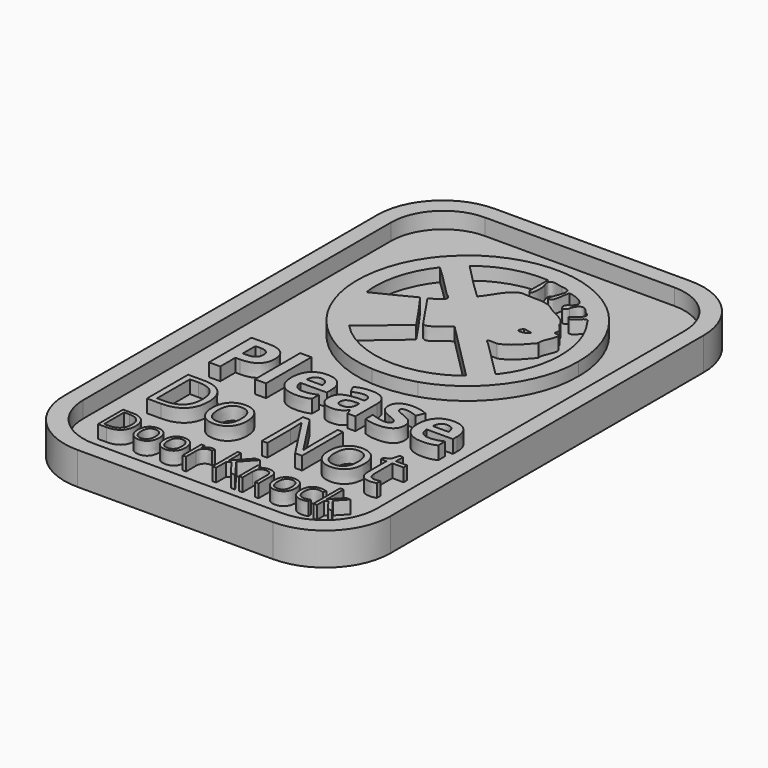
from build123d import *

# Parameters (mm, degrees)
F0_W           = 50
F0_H           = 25
F0_H_2         = 55
F1_DEPTH       = 5
F2_T           = -2.5
F3_TEXT_SIZE   = 11.4280198832
F3_TEXT_SIZE_2 = 11.0519929058
F3_TEXT_SIZE_3 = 6.7370337705
F4_DEPTH       = 2
F5_R           = 8
F6_R           = 10
F8_DEPTH       = 2


# Not quite as in the source:
# - ends of sketch curves that miss each other by under 0.0002 mm in the source are joined
# - Text() gives the source's letters only with a copy of the font that has no kerning and outlines rounded to 1/6400 em; it was checked with that copy


with BuildPart() as f1:
    # F0 (on Top) → F1 (new body)
    with BuildSketch(Plane.XY):
        with Locations((0, 12.5)):
            Rectangle(F0_W, F0_H)
        with Locations((0, -27.5)):
            Rectangle(F0_W, F0_H_2)
    extrude(amount=F1_DEPTH)

    # F2
    f2_openings = [f1.faces().sort_by_distance(p)[0] for p in [
        (0, -15, 5),
    ]]
    offset(amount=F2_T, openings=f2_openings)

    # F3 (on face) → F4 (join)
    with BuildSketch(Plane.XY.offset(2.5)):
        with Locations((-18.5, -26.691900793)):
            Text('Please', F3_TEXT_SIZE, font='Open Sans', font_style=FontStyle.BOLD, text_align=(TextAlign.LEFT, TextAlign.BOTTOM))
        with Locations((-18.5, -38.6493356852)):
            Text('Do Not', F3_TEXT_SIZE_2, font='Open Sans', text_align=(TextAlign.LEFT, TextAlign.BOTTOM))
        with Locations((-18.5, -47.5)):
            Text('Door Knock', F3_TEXT_SIZE_3, font='Open Sans', text_align=(TextAlign.LEFT, TextAlign.BOTTOM))
    extrude(amount=F4_DEPTH)

    # F5
    f5_edges = [f1.edges().sort_by_distance(p)[0] for p in [
        (-22.5, 22.5, 3.75),
        (22.5, 22.5, 3.75),
        (22.5, -52.5, 3.75),
        (-22.5, -52.5, 3.75),
    ]]
    fillet(f5_edges, radius=F5_R)

    # F6
    f6_edges = [f1.edges().sort_by_distance(p)[0] for p in [
        (-25, 25, 2.5),
        (-25, -55, 2.5),
        (25, -55, 2.5),
        (25, 25, 2.5),
    ]]
    fillet(f6_edges, radius=F6_R)

    # F7 (on face) → F8 (join)
    with BuildSketch(Plane.XY.offset(2.5)):
        with BuildLine():
            add(Edge.make_bspline(
                [(-1.152975, -15.828035), (-7.683402, -15.45201), (-13.720566, -10.924744), (-15.897689, -4.754124)],
                knots=[0, 0, 0, 0, 1, 1, 1, 1], degree=3))
            add(Edge.make_bspline(
                [(5.254472, -15.031673), (3.193987, -15.71671), (1.009548, -15.937421), (-1.152975, -15.828035)],
                knots=[0, 0, 0, 0, 1, 1, 1, 1], degree=3))
            add(Edge.make_bspline(
                [(16.918267, 1.099339), (17.077182, -6.063448), (12.07656, -12.904762), (5.254472, -15.031673)],
                knots=[0, 0, 0, 0, 1, 1, 1, 1], degree=3))
            add(Edge.make_bspline(
                [(6.093725, 16.862866), (12.482614, 14.48419), (17.023863, 7.927673), (16.918267, 1.099339)],
                knots=[0, 0, 0, 0, 1, 1, 1, 1], degree=3))
            add(Edge.make_bspline(
                [(-12.087027, 12.911491), (-7.523079, 17.697854), (-0.044603, 19.290758), (6.093725, 16.862866)],
                knots=[0, 0, 0, 0, 1, 1, 1, 1], degree=3))
            add(Edge.make_bspline(
                [(-15.897689, -4.754124), (-18.132821, 1.226539), (-16.624786, 8.400491), (-12.087027, 12.911491)],
                knots=[0, 0, 0, 0, 1, 1, 1, 1], degree=3))
        make_face()
        with BuildLine():
            add(Edge.make_bspline(
                [(1.660306, -13.112709), (4.218505, -12.787149), (6.73921, -11.822528), (8.738555, -10.17936)],
                knots=[0, 0, 0, 0, 1, 1, 1, 1], degree=3))
            add(Edge.make_bspline(
                [(-10.297667, -8.802453), (-7.267469, -12.026995), (-2.724918, -13.624278), (1.660306, -13.112709)],
                knots=[0, 0, 0, 0, 1, 1, 1, 1], degree=3))
            add(Edge.make_bspline(
                [(-4.186312, -3.599084), (-6.159197, -5.403336), (-8.265193, -7.063118), (-10.297667, -8.802453)],
                knots=[0, 0, 0, 0, 1, 1, 1, 1], degree=3))
            add(Edge.make_bspline(
                [(-8.239712, 2.231822), (-6.846707, 0.318469), (-5.495582, -1.627468), (-4.186312, -3.599084)],
                knots=[0, 0, 0, 0, 1, 1, 1, 1], degree=3))
            add(Edge.make_bspline(
                [(-14.12669, -0.727469), (-12.153893, 0.147058), (-10.217288, 1.29033), (-8.239712, 2.231822)],
                knots=[0, 0, 0, 0, 1, 1, 1, 1], degree=3))
            add(Edge.make_bspline(
                [(-11.252573, 9.780323), (-13.58058, 6.880246), (-14.657997, 2.956887), (-14.12669, -0.727469)],
                knots=[0, 0, 0, 0, 1, 1, 1, 1], degree=3))
            add(Edge.make_bspline(
                [(-6.241496, 4.836455), (-7.914058, 6.474699), (-9.527901, 8.223918), (-11.252573, 9.780323)],
                knots=[0, 0, 0, 0, 1, 1, 1, 1], degree=3))
            add(Edge.make_bspline(
                [(-7.363937, 2.526994), (-6.492223, 3.287102), (-4.519532, 3.854826), (-6.241496, 4.836455)],
                knots=[0, 0, 0, 0, 1, 1, 1, 1], degree=3))
            add(Edge.make_bspline(
                [(-3.768493, -2.787968), (-4.965583, -1.015428), (-6.195906, 0.735116), (-7.363937, 2.526994)],
                knots=[0, 0, 0, 0, 1, 1, 1, 1], degree=3))
            add(Edge.make_bspline(
                [(-0.275679, -1.122884), (-1.382058, -1.544562), (-2.812765, -3.748359), (-3.768493, -2.787968)],
                knots=[0, 0, 0, 0, 1, 1, 1, 1], degree=3))
            add(Edge.make_bspline(
                [(8.738555, -10.17936), (5.763579, -7.131316), (2.730646, -4.140094), (-0.275679, -1.122884)],
                knots=[0, 0, 0, 0, 1, 1, 1, 1], degree=3))
        make_face(mode=Mode.SUBTRACT)
        with BuildLine():
            add(Edge.make_bspline(
                [(6.601974, 3.609834), (5.43198, 2.241723), (7.786639, 2.813194), (7.906053, 3.364306)],
                knots=[0, 0, 0, 0, 1, 1, 1, 1], degree=3))
            add(Edge.make_bspline(
                [(7.906053, 3.364306), (7.469209, 3.433762), (7.043806, 3.588845), (6.601974, 3.609834)],
                knots=[0, 0, 0, 0, 1, 1, 1, 1], degree=3))
        make_face(mode=Mode.SUBTRACT)
        with BuildLine():
            add(Edge.make_bspline(
                [(11.485483, -7.404762), (15.186964, -2.533407), (15.184399, 4.740779), (11.442712, 9.589734)],
                knots=[0, 0, 0, 0, 1, 1, 1, 1], degree=3))
            Line((11.485483, -7.404762), (11.241475, -7.677406))
            add(Edge.make_bspline(
                [(5.496094, -1.966448), (7.401659, -3.879546), (9.301033, -5.799784), (11.241475, -7.677406)],
                knots=[0, 0, 0, 0, 1, 1, 1, 1], degree=3))
            add(Edge.make_bspline(
                [(6.395967, -1.373541), (5.665343, -1.359618), (4.317876, -1.147458), (5.496094, -1.966448)],
                knots=[0, 0, 0, 0, 1, 1, 1, 1], degree=3))
            add(Edge.make_bspline(
                [(10.203608, 1.80601), (9.183774, 0.601692), (7.949414, -0.912305), (6.395967, -1.373541)],
                knots=[0, 0, 0, 0, 1, 1, 1, 1], degree=3))
            add(Edge.make_bspline(
                [(10.044016, 5.036102), (12.119685, 5.22382), (9.807728, 2.933683), (10.203608, 1.80601)],
                knots=[0, 0, 0, 0, 1, 1, 1, 1], degree=3))
            add(Edge.make_bspline(
                [(9.0461, 7.518678), (9.156834, 6.566266), (10.609032, 6.326291), (10.044016, 5.036102)],
                knots=[0, 0, 0, 0, 1, 1, 1, 1], degree=3))
            add(Edge.make_bspline(
                [(5.483761, 10.010437), (6.569352, 9.043758), (8.258383, 8.793305), (9.0461, 7.518678)],
                knots=[0, 0, 0, 0, 1, 1, 1, 1], degree=3))
            add(Edge.make_bspline(
                [(0.600075, 10.698445), (2.204529, 10.477569), (4.073608, 10.895719), (5.483761, 10.010437)],
                knots=[0, 0, 0, 0, 1, 1, 1, 1], degree=3))
            add(Edge.make_bspline(
                [(-3.082797, 6.690972), (-1.847459, 7.993295), (-1.247836, 10.197991), (0.600075, 10.698445)],
                knots=[0, 0, 0, 0, 1, 1, 1, 1], degree=3))
            add(Edge.make_bspline(
                [(-8.70876, 12.289), (-6.870993, 10.388065), (-5.026789, 8.480831), (-3.082797, 6.690972)],
                knots=[0, 0, 0, 0, 1, 1, 1, 1], degree=3))
            add(Edge.make_bspline(
                [(0.918824, 15.289045), (-2.491031, 15.510739), (-6.082567, 14.509325), (-8.70876, 12.289)],
                knots=[0, 0, 0, 0, 1, 1, 1, 1], degree=3))
            add(Edge.make_bspline(
                [(0.876587, 11.922761), (0.890665, 13.044855), (0.904744, 14.166951), (0.918824, 15.289045)],
                knots=[0, 0, 0, 0, 1, 1, 1, 1], degree=3))
            add(Edge.make_bspline(
                [(1.408202, 14.041427), (1.783509, 13.249301), (1.537262, 10.237396), (0.876587, 11.922761)],
                knots=[0, 0, 0, 0, 1, 1, 1, 1], degree=3))
            add(Edge.make_bspline(
                [(3.287114, 14.952799), (2.264517, 15.218973), (0.734889, 15.722643), (1.408202, 14.041427)],
                knots=[0, 0, 0, 0, 1, 1, 1, 1], degree=3))
            add(Edge.make_bspline(
                [(3.784854, 11.639946), (3.996849, 12.895314), (5.639773, 15.041058), (3.287114, 14.952799)],
                knots=[0, 0, 0, 0, 1, 1, 1, 1], degree=3))
            add(Edge.make_bspline(
                [(5.049218, 14.2195), (4.740171, 13.412628), (4.881133, 10.926293), (3.784854, 11.639946)],
                knots=[0, 0, 0, 0, 1, 1, 1, 1], degree=3))
            add(Edge.make_bspline(
                [(7.038289, 11.838488), (8.903538, 13.118997), (5.965443, 14.197563), (5.049218, 14.2195)],
                knots=[0, 0, 0, 0, 1, 1, 1, 1], degree=3))
            add(Edge.make_bspline(
                [(7.497503, 11.19198), (7.161075, 9.770424), (5.861606, 11.256564), (7.038289, 11.838488)],
                knots=[0, 0, 0, 0, 1, 1, 1, 1], degree=3))
            add(Edge.make_bspline(
                [(9.607956, 11.610006), (8.729716, 12.835495), (7.899914, 12.607578), (7.497503, 11.19198)],
                knots=[0, 0, 0, 0, 1, 1, 1, 1], degree=3))
            add(Edge.make_bspline(
                [(8.799988, 9.365286), (9.603146, 10.056716), (11.148793, 10.801712), (9.607956, 11.610006)],
                knots=[0, 0, 0, 0, 1, 1, 1, 1], degree=3))
            add(Edge.make_bspline(
                [(11.442712, 9.589734), (10.728221, 11.531846), (9.632121, 7.908508), (8.799988, 9.365286)],
                knots=[0, 0, 0, 0, 1, 1, 1, 1], degree=3))
        make_face(mode=Mode.SUBTRACT)
    extrude(amount=F8_DEPTH)


solid = f1.part
